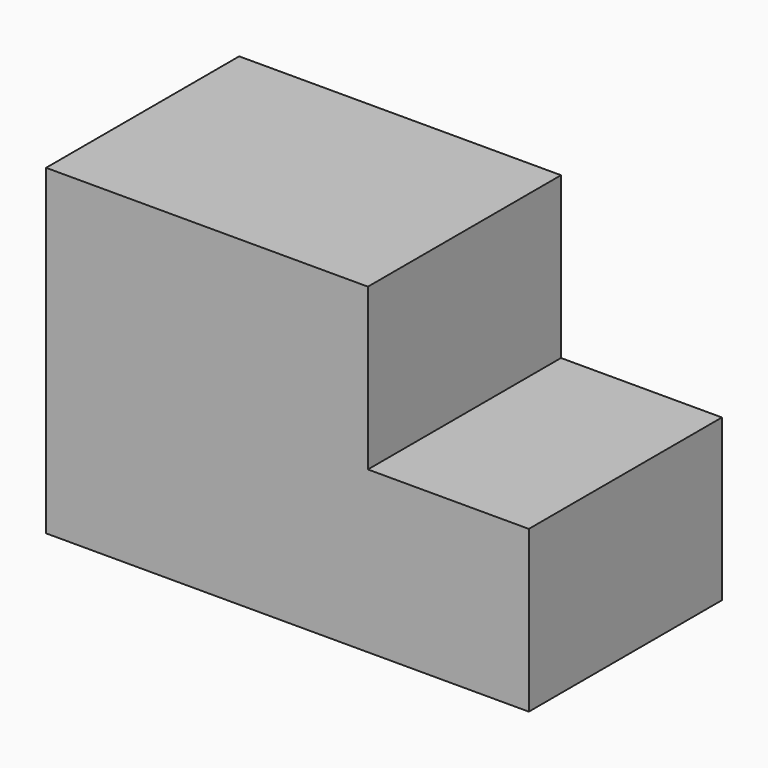
from build123d import *

# Parameters (mm, degrees)
F7_DEPTH = 38.1


# Not quite as in the source:
# - a feature of the source that left no trace in its solid (it failed there, or was rolled back) is left out


with BuildPart() as f7:
    # F6 (on Front) → F7 (new body)
    with BuildSketch(Plane.XZ):
        Polygon((-36.6813843086, 22.1439363986), (-36.6813843086, -28.6560636014), (39.5186156914, -28.6560636014), (39.5186156914, -3.2560636014), (14.1186156914, -3.2560636014), (14.1186156914, 22.1439363986), align=None)
    extrude(amount=F7_DEPTH)


solid = f7.part
